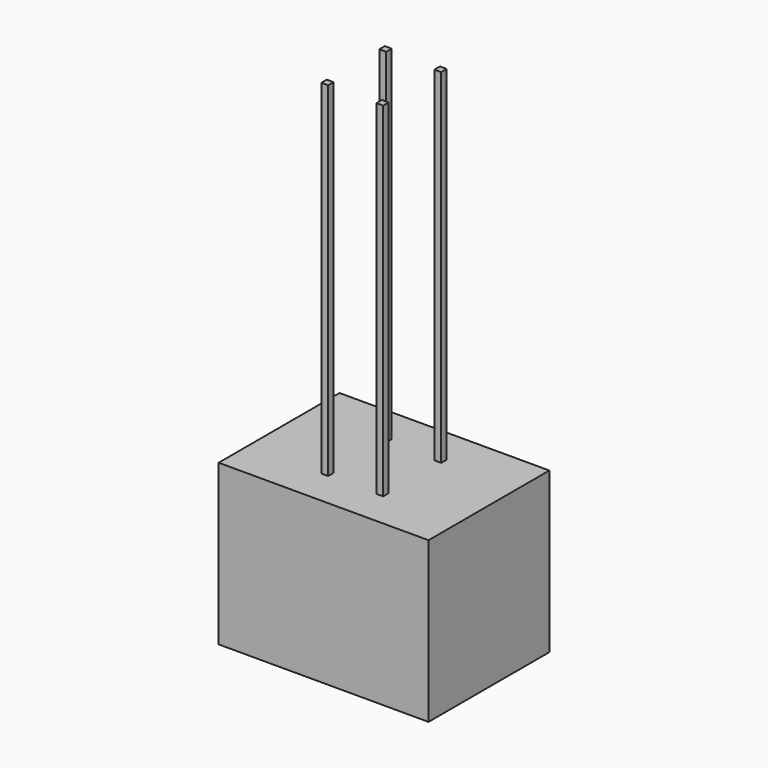
from build123d import *

# Parameters (mm, degrees)
F0_W     = 6.1
F0_H     = 4.65
F1_DEPTH = 2.195
F3_W     = 0.2
F3_H     = 0.2
F4_DEPTH = 10


# Not quite as in the source:
# - a feature of the source that left no trace in its solid (it failed there, or was rolled back) is left out


with BuildPart() as f1:
    # F0 (on Front) → F1 (new body, symmetric)
    with BuildSketch(Plane.XZ):
        Rectangle(F0_W, F0_H)
    extrude(amount=F1_DEPTH, both=True)

    # F3 (on face) → F4 (join)
    with BuildSketch(Plane.XY.offset(2.325)):
        with Locations((0.8, 1.055)):
            Rectangle(F3_W, F3_H)
        with Locations((-0.8, 1.055)):
            Rectangle(F3_W, F3_H)
        with Locations((0.8, -1.055)):
            Rectangle(F3_W, F3_H)
        with Locations((-0.8, -1.055)):
            Rectangle(F3_W, F3_H)
    extrude(amount=F4_DEPTH)


solid = f1.part
